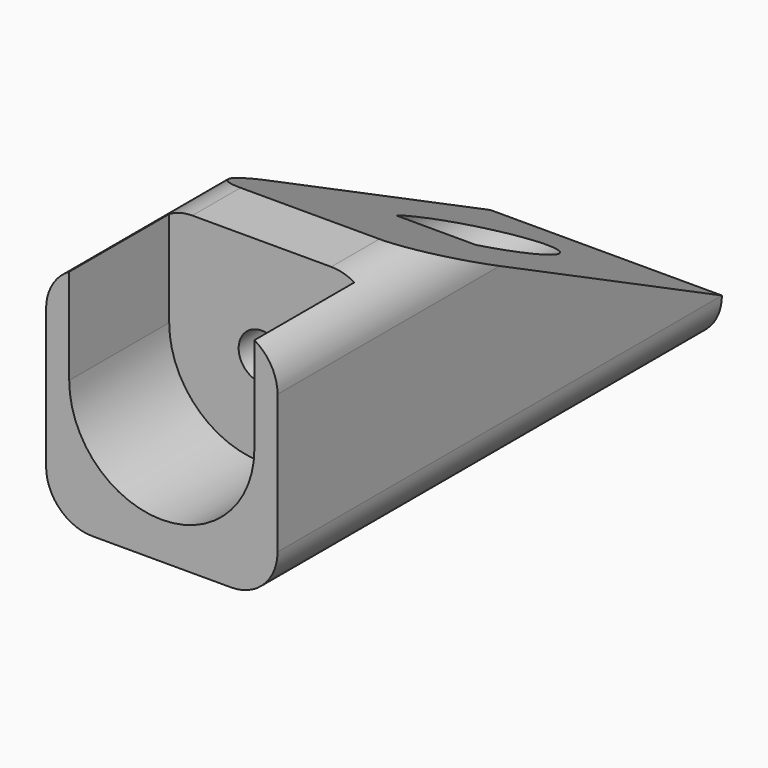
from build123d import *

# Parameters (mm, degrees)
F0_W        = 25
F0_H        = 60
F1_DEPTH    = 25
F2_R        = 5
F4_DEPTH    = 13.5
F5_DEPTH    = 13.5
F6_T1_DEPTH = 222.1863099029
F7_R        = 2.5
F8_DEPTH    = 55
F10_START   = -23.5
F9_R        = 5
F10_DEPTH   = 23


# Not quite as in the source:
# - a fillet or chamfer that OpenCascade refuses, or shapes differently, is made with other operations: its cross-section is extruded or revolved along the edge and cut away or added
# - ends of sketch curves that miss each other by under 0.0002 mm in the source are joined


with BuildPart() as f1:
    # F0 (on Top) → F1 (new body)
    with BuildSketch(Plane.XY):
        Rectangle(F0_W, F0_H)
    extrude(amount=F1_DEPTH)

    # F2
    f2_edges = [f1.edges().sort_by_distance(p)[0] for p in [
        (12.5, 0, 25),
        (12.5, 0, 0),
        (-12.5, 0, 0),
        (-12.5, 0, 25),
    ]]
    fillet(f2_edges, radius=F2_R)

    # F3 (on face) → F4 (cut)
    with BuildSketch(Plane.XZ.offset(30)):
        with BuildLine():
            Line((-10, 13.9999993678), (10, 13.9999993678))
            ThreePointArc((10, 13.9999993678), (-3.161e-07, 24), (-10, 13.9999993678))
        make_face()
        with BuildLine():
            ThreePointArc((-10, 13.9999993678), (3.161e-07, 4), (10, 14))
            Line((10, 14), (-10, 13.9999993678))
        make_face()
    extrude(amount=-F4_DEPTH, mode=Mode.SUBTRACT)

    # F3 (on face) → F5 (cut)
    with BuildSketch(Plane.XZ.offset(30)):
        with BuildLine():
            ThreePointArc((-10, 13.9999993678), (-3.161e-07, 24), (10, 14))
            Line((10, 14), (10, 24.3301270189))
            ThreePointArc((10, 24.3301270189), (8.7940952255, 24.8296291314), (7.5, 25))
            Line((7.5, 25), (-7.5, 25))
            ThreePointArc((-7.5, 25), (-8.7940952255, 24.8296291314), (-10, 24.3301270189))
            Line((-10, 24.3301270189), (-10, 13.9999993678))
        make_face()
    extrude(amount=-F5_DEPTH, mode=Mode.SUBTRACT)

    # F6: chamfer of 40 x 20 on 1 edges, made by hand

    # F6_s2 → F6_t1 (cut)
    with BuildSketch(Plane.YZ.offset(-111.0931549515)):
        Polygon((30, 5), (-10, 25), (30, 25), align=None)
    extrude(amount=F6_T1_DEPTH, mode=Mode.SUBTRACT)

    # F7 (on face) → F8 (cut)
    with BuildSketch(Plane.XZ.offset(16.5)):
        with Locations((0, 14)):
            Circle(F7_R)
    extrude(amount=-F8_DEPTH, mode=Mode.SUBTRACT)

    # F9 (on face) → F10 (cut)
    with BuildSketch(Plane.XZ.offset(16.5).offset(F10_START)):
        with Locations((0, 14)):
            Circle(F9_R)
    extrude(amount=-F10_DEPTH, mode=Mode.SUBTRACT)


solid = f1.part
